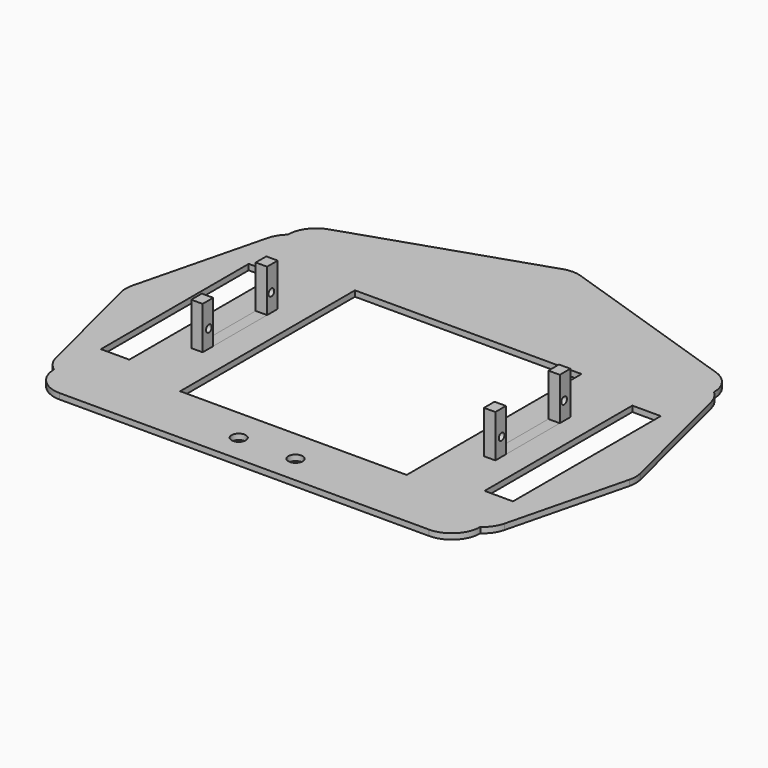
from build123d import *

# Parameters (mm, degrees)
F0_R         = 2.5
F0_W         = 10
F0_H         = 65
F1_DEPTH     = 2
F2_DEPTH     = 15
F3_R         = 10
F4_R         = 1.25
F5_DEPTH     = 4.4
F6_DEPTH     = 2
F7_R         = 1.25
F8_DEPTH     = 4.7
F7_W         = 23.7
F7_H         = 15
F9_DEPTH     = 4.3
F10_DEPTH    = 2
F11_T1_DEPTH = 83.1509498697
F11_T3_DEPTH = 65.2047050598
F11_T5_DEPTH = 14.5


# Not quite as in the source:
# - a fillet or chamfer that OpenCascade refuses, or shapes differently, is made with other operations: its cross-section is extruded or revolved along the edge and cut away or added


with BuildPart() as f1:
    # F0 (on Top) → F1 (new body)
    with BuildSketch(Plane.XY):
        Polygon((0, 85), (-75, 60), (0, 60), align=None)
        Polygon((0, 85), (0, 60), (75, 60), align=None)
        Polygon((0, 60), (-75, 60), (-75, -60), (0, -60), (75, -60), (75, 60), align=None)
        with Locations((-10, -50)):
            Circle(F0_R, mode=Mode.SUBTRACT)
        with Locations((-67.5, 0)):
            Rectangle(F0_W, F0_H, mode=Mode.SUBTRACT)
        Polygon((-53.5, 16.5), (-49.5, 16.5), (-49.5, 12), (-49.5, -12), (-49.5, -16.5), (-53.5, -16.5), align=None, mode=Mode.SUBTRACT)
        with Locations((10, -50)):
            Circle(F0_R, mode=Mode.SUBTRACT)
        Polygon((39.8586168885, -38.4434349835), (0, -38.4434349835), (-39.8586168885, -38.4434349835), (-39.8586168885, 38.4434349835), (39.8586168885, 38.4434349835), align=None, mode=Mode.SUBTRACT)
        Polygon((49.5, 12), (49.5, 16.5), (53.5, 16.5), (53.5, -16.5), (49.5, -16.5), (49.5, -12), align=None, mode=Mode.SUBTRACT)
        with Locations((67.5, 0)):
            Rectangle(F0_W, F0_H, mode=Mode.SUBTRACT)
    extrude(amount=-F1_DEPTH)

    # F3
    f3_edges = [f1.edges().sort_by_distance(p)[0] for p in [
        (-75, -60, -1),
        (75, -60, -1),
        (75, 60, -1),
        (0, 85, -1),
        (-75, 60, -1),
    ]]
    fillet(f3_edges, radius=F3_R)

    # F0 (on Top) → F10 (join)
    with BuildSketch(Plane.XY):
        Polygon((-75, -60), (-75, 60), (-90, 0), align=None)
        Polygon((90, 0), (75, 60), (75, -60), align=None)
    extrude(amount=-F10_DEPTH)

    # F11: fillet of radius 10 on 6 edges, made by hand

    # F11_s2 → F11_t1 (cut)
    with BuildSketch(Plane.XY.offset(-42.5754749349)):
        with BuildLine():
            ThreePointArc((-75, -50), (-77.484564926, -47.4809714737), (-78.9363992698, -44.2544029208))
            Line((-78.9363992698, -44.2544029208), (-75, -60))
            Line((-75, -60), (-75, -50))
        make_face()
        with BuildLine():
            ThreePointArc((75, -50), (77.484564926, -47.4809714737), (78.9363992698, -44.2544029208))
            Line((78.9363992698, -44.2544029208), (75, -60))
            Line((75, -60), (75, -50))
        make_face()
    extrude(amount=F11_T1_DEPTH, mode=Mode.SUBTRACT)

    # F11_s4 → F11_t3 (cut)
    with BuildSketch(Plane.XY.offset(-33.6023525299)):
        with BuildLine():
            ThreePointArc((75, 52.7924077994), (76.9151696289, 50.4962288752), (78.0658785294, 47.7364858825))
            Line((78.0658785294, 47.7364858825), (75, 60))
            Line((75, 60), (75, 52.7924077994))
        make_face()
        with BuildLine():
            ThreePointArc((-75, 52.7924077994), (-76.9151696289, 50.4962288752), (-78.0658785294, 47.7364858825))
            Line((-78.0658785294, 47.7364858825), (-75, 60))
            Line((-75, 60), (-75, 52.7924077994))
        make_face()
    extrude(amount=F11_T3_DEPTH, mode=Mode.SUBTRACT)

    # F11_s6 → F11_t5 (cut)
    with BuildSketch(Plane.XY.offset(-8.25)):
        with BuildLine():
            ThreePointArc((89.3936609374, 2.4253562504), (89.692235936, 0), (89.3936609374, -2.4253562504))
            Line((89.3936609374, -2.4253562504), (90, 0))
            Line((90, 0), (89.3936609374, 2.4253562504))
        make_face()
        with BuildLine():
            ThreePointArc((-89.3936609374, -2.4253562504), (-89.692235936, 0), (-89.3936609374, 2.4253562504))
            Line((-89.3936609374, 2.4253562504), (-90, 0))
            Line((-90, 0), (-89.3936609374, -2.4253562504))
        make_face()
    extrude(amount=F11_T5_DEPTH, mode=Mode.SUBTRACT)


with BuildPart() as f2:
    # F0 (on Top) → F2 (new body)
    with BuildSketch(Plane.XY):
        Polygon((-49.5, 12), (-49.5, 16.5), (-53.5, 16.5), (-53.5, -16.5), (-49.5, -16.5), (-49.5, -12), align=None)
    extrude(amount=F2_DEPTH)

    # F4 (on face) → F5 (cut)
    with BuildSketch(Plane(origin=(-53.5, 0, 0), x_dir=(0, -1, 0), z_dir=(-1, 0, 0))):
        with Locations((-13.75, 6.25)):
            Circle(F4_R)
        with Locations((13.75, 6.25)):
            Circle(F4_R)
        Polygon((11.85, 15), (0, 15), (-11.85, 15), (-11.85, 0), (11.85, 0), align=None)
    extrude(amount=-F5_DEPTH, mode=Mode.SUBTRACT)


with BuildPart() as f2b:
    # F0 (on Top) → F2, piece 2 (new body)
    with BuildSketch(Plane.XY):
        Polygon((53.5, 16.5), (49.5, 16.5), (49.5, 12), (49.5, -12), (49.5, -16.5), (53.5, -16.5), align=None)
    extrude(amount=F2_DEPTH)

    # F7 (on face) → F8 (cut)
    with BuildSketch(Plane(origin=(49.5, 0, 0), x_dir=(0, -1, 0), z_dir=(-1, 0, 0))):
        with Locations((-13.75, 6.25)):
            Circle(F7_R)
        with Locations((13.75, 6.25)):
            Circle(F7_R)
    extrude(amount=-F8_DEPTH, mode=Mode.SUBTRACT)

    # F7 (on face) → F9 (cut)
    with BuildSketch(Plane(origin=(49.5, 0, 0), x_dir=(0, -1, 0), z_dir=(-1, 0, 0))):
        with Locations((0, 7.5)):
            Rectangle(F7_W, F7_H)
    extrude(amount=-F9_DEPTH, mode=Mode.SUBTRACT)


with BuildPart() as f6:
    # F0 (on Top) → F6 (new body)
    with BuildSketch(Plane.XY):
        Polygon((53.5, 16.5), (49.5, 16.5), (49.5, 12), (49.5, -12), (49.5, -16.5), (53.5, -16.5), align=None)
    extrude(amount=-F6_DEPTH)


with BuildPart() as f6b:
    # F0 (on Top) → F6, piece 2 (new body)
    with BuildSketch(Plane.XY):
        Polygon((-49.5, 12), (-49.5, 16.5), (-53.5, 16.5), (-53.5, -16.5), (-49.5, -16.5), (-49.5, -12), align=None)
    extrude(amount=-F6_DEPTH)


solid = Compound([f1.part, f2.part, f2b.part, f6.part, f6b.part])
